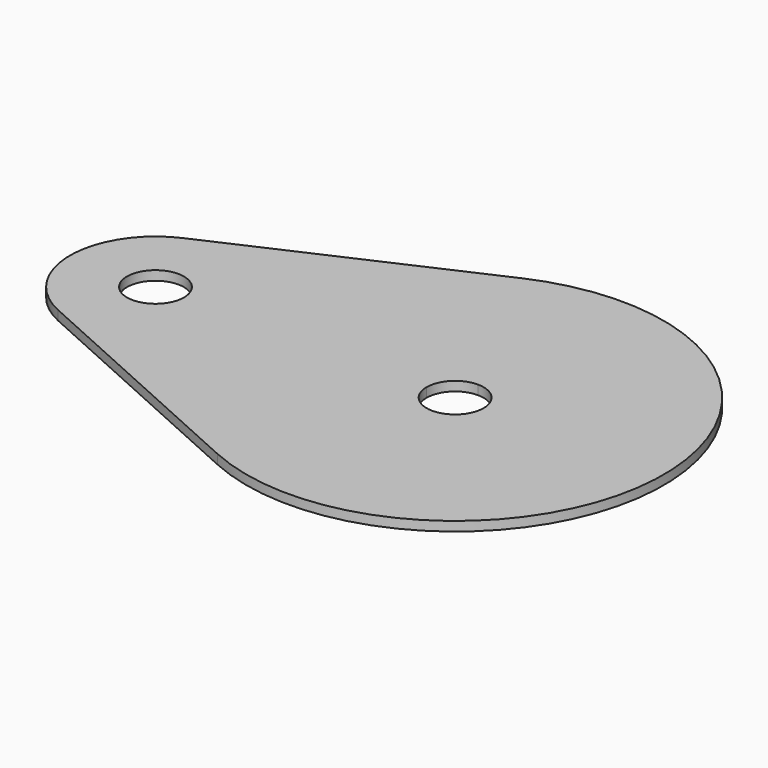
from build123d import *

# Parameters (mm, degrees)
F0_R     = 13.9065
F0_R_2   = 9.652
F1_DEPTH = 3.175


# Not quite as in the source:
# - a length typed as a fraction of an inch, garbled in the dataset ("3 / 203.2 mm" for 3/8 in), is restored


with BuildPart() as f1:
    # F0 (on Top) → F1 (new body)
    with BuildSketch(Plane.XY):
        with BuildLine():
            Line((-29.0468705796, 64.4645603781), (-113.5004093806, 26.4109228888))
            ThreePointArc((-113.5004093806, 26.4109228888), (-130.5681996552, 0), (-113.5004093806, -26.4109228888))
            Line((-113.5004093806, -26.4109228888), (-29.0468705796, -64.4645603781))
            ThreePointArc((-29.0468705796, -64.4645603781), (70.706437014, 0), (-29.0468705796, 64.4645603781))
        make_face()
        with Locations((-101.6, 0)):
            Circle(F0_R, mode=Mode.SUBTRACT)
        with BuildLine():
            ThreePointArc((0, 64.77), (45.7993062175, 45.7993062175), (64.77, 0))
            ThreePointArc((64.77, 0), (45.7993062175, -45.7993062175), (0, -64.77))
            ThreePointArc((0, -64.77), (-45.7993062175, -45.7993062175), (-64.77, 0))
            ThreePointArc((-64.77, 0), (-45.7993062175, 45.7993062175), (0, 64.77))
        make_face(mode=Mode.SUBTRACT)
        with Locations((-101.6, 0)):
            Circle(F0_R)
        with Locations((-101.6, 0)):
            Circle(F0_R_2, mode=Mode.SUBTRACT)
        with BuildLine():
            Line((0, 9.652), (0, 64.77))
            ThreePointArc((0, 64.77), (-45.7993062175, 45.7993062175), (-64.77, 0))
            Line((-64.77, 0), (-9.652, 0))
            ThreePointArc((-9.652, 0), (-6.824994652, 6.824994652), (0, 9.652))
        make_face()
        with BuildLine():
            ThreePointArc((-64.77, 0), (-45.7993062175, -45.7993062175), (0, -64.77))
            Line((0, -64.77), (0, -9.652))
            ThreePointArc((0, -9.652), (-6.824994652, -6.824994652), (-9.652, 0))
            Line((-9.652, 0), (-64.77, 0))
        make_face()
        with BuildLine():
            ThreePointArc((0, -64.77), (45.7993062175, -45.7993062175), (64.77, 0))
            ThreePointArc((64.77, 0), (45.7993062175, 45.7993062175), (0, 64.77))
            Line((0, 64.77), (0, 9.652))
            ThreePointArc((0, 9.652), (6.824994652, 6.824994652), (9.652, 0))
            ThreePointArc((9.652, 0), (6.824994652, -6.824994652), (0, -9.652))
            Line((0, -9.652), (0, -64.77))
        make_face()
    extrude(amount=F1_DEPTH)


solid = f1.part
